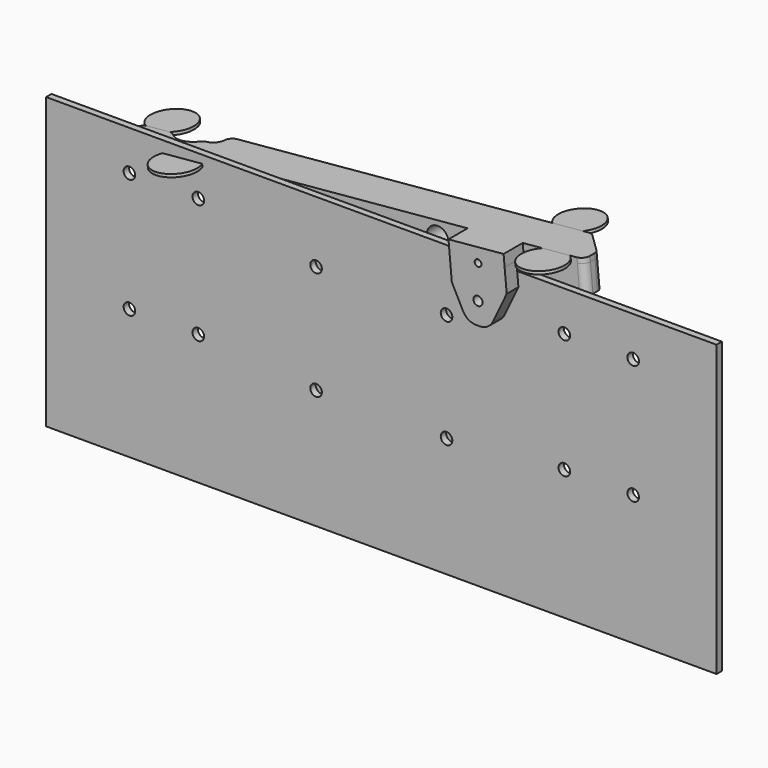
from build123d import *

# Parameters (mm, degrees)
F0_R          = 1.5875
F1_DEPTH      = 15.24
F1_DEPTH_BACK = 7.62
F2_DEPTH      = 2.4892
F3_DEPTH      = 25.4
F3_DEPTH_BACK = 0.762
F4_R          = 5.08
F5_R          = 1.7705235874
F6_DEPTH      = 26.9611633365
F7_W          = 234.95
F7_H          = 101.6
F7_R          = 2.032
F7_R_2        = 1.651
F8_DEPTH      = 2.3622
F10_DEPTH     = 114.7801239931
F11_W         = 54.61
F11_H         = 50.8
F12_DEPTH     = 25.4
F14_R         = 1.7705235874
F15_DEPTH     = 25.4
F16_R         = 3.302
F17_DEPTH     = 25.4
F18_SIZE      = 8.89
F19_R         = 1.1811
F20_DEPTH     = 48.26
F21_T4_DEPTH  = 12.1179471252
F21_S5_R      = 1.1811
F21_T6_DEPTH  = 8
F21_T11_DEPTH = 12.1179471252
F21_S12_R     = 1.1811
F21_T13_DEPTH = 8
F22_R         = 2.54
F23_R         = 7.62
F24_DEPTH     = 1.016
F25_R         = 3.7728074262
F25_R_2       = 2.7641232058
F26_DEPTH     = 28.2579587291


# Not quite as in the source:
# - a fillet or chamfer that OpenCascade refuses, or shapes differently, is made with other operations: its cross-section is extruded or revolved along the edge and cut away or added


with BuildPart() as f1:
    # F0 (on Front) → F1 (new body, two sides)
    with BuildSketch(Plane.XZ) as f1_sk:
        Polygon((-9.9150021419, 10.8382269042), (-131.9738921994, 3.3727853757), (-131.6879499686, 0.2364539576), (-9.1841964381, 2.8224508396), align=None)
        Polygon((-10.3522961262, 15.6346462997), (-132.08, 4.5366191606), (-131.9738921994, 3.3727853757), (-9.9150021419, 10.8382269042), align=None)
        Polygon((8.9584602173, 17.3952257829), (-10.3522961262, 15.6346462997), (-9.9150021419, 10.8382269042), (-0.3070324239, 11.4258755065), (9.3269835997, 13.3531104945), align=None)
        Polygon((-0.3070324239, 11.4258755065), (-9.9150021419, 10.8382269042), (-9.1841964381, 2.8224508396), (-3.81, -7.62), (3.81, -7.62), (10.047620121, 5.4488741869), (9.3269835997, 13.3531104945), align=None)
        Circle(F0_R, mode=Mode.SUBTRACT)
        Polygon((30.6387240807, 17.6164137534), (9.3269835997, 13.3531104945), (10.047620121, 5.4488741869), (31.5177794949, 7.97457419), align=None)
        Polygon((30.48, 19.3573644332), (8.9584602173, 17.3952257829), (9.3269835997, 13.3531104945), (30.6387240807, 17.6164137534), align=None)
    extrude(amount=-F1_DEPTH)
    extrude(f1_sk.sketch, amount=F1_DEPTH_BACK)

    # F0 (on Front) → F2 (cut)
    with BuildSketch(Plane.XZ):
        Polygon((-9.9150021419, 10.8382269042), (-131.9738921994, 3.3727853757), (-131.6879499686, 0.2364539576), (-9.1841964381, 2.8224508396), align=None)
        Polygon((-0.3070324239, 11.4258755065), (-9.9150021419, 10.8382269042), (-9.1841964381, 2.8224508396), (-3.81, -7.62), (3.81, -7.62), (10.047620121, 5.4488741869), (9.3269835997, 13.3531104945), align=None)
        Circle(F0_R, mode=Mode.SUBTRACT)
        Polygon((30.6387240807, 17.6164137534), (9.3269835997, 13.3531104945), (10.047620121, 5.4488741869), (31.5177794949, 7.97457419), align=None)
    extrude(amount=F2_DEPTH, mode=Mode.SUBTRACT)

    # F0 (on Front) → F3 (cut, two sides)
    with BuildSketch(Plane.XZ) as f3_sk:
        Polygon((-9.9150021419, 10.8382269042), (-131.9738921994, 3.3727853757), (-131.6879499686, 0.2364539576), (-9.1841964381, 2.8224508396), align=None)
        Polygon((-10.3522961262, 15.6346462997), (-132.08, 4.5366191606), (-131.9738921994, 3.3727853757), (-9.9150021419, 10.8382269042), align=None)
        Polygon((30.6387240807, 17.6164137534), (9.3269835997, 13.3531104945), (10.047620121, 5.4488741869), (31.5177794949, 7.97457419), align=None)
        Polygon((30.48, 19.3573644332), (8.9584602173, 17.3952257829), (9.3269835997, 13.3531104945), (30.6387240807, 17.6164137534), align=None)
    extrude(amount=F3_DEPTH, mode=Mode.SUBTRACT)
    extrude(f3_sk.sketch, amount=-F3_DEPTH_BACK, mode=Mode.SUBTRACT)

    # F4
    f4_edges = [f1.edges().sort_by_distance(p)[0] for p in [
        (-3.81, 7.62, -7.62),
        (-3.81, -5.0546, -7.62),
        (3.81, -5.0546, -7.62),
        (3.81, 7.62, -7.62),
    ]]
    fillet(f4_edges, radius=F4_R)

    # F5 (on face) → F6 (cut, through all)
    with BuildSketch(Plane(origin=(-1.4990148259, 0, 16.441808129), x_dir=(0.9958696626, 0, 0.0907943565), z_dir=(-0.0907943565, 0, 0.9958696626))):
        with Locations((-124.7725656148, 5.08)):
            Circle(F5_R)
    extrude(amount=-F6_DEPTH, mode=Mode.SUBTRACT)

    # F9 (on face) → F10 (cut, through all)
    with BuildSketch(Plane(origin=(-1.4990148259, 0, 16.441808129), x_dir=(0.9958696626, 0, 0.0907943565), z_dir=(-0.0907943565, 0, 0.9958696626))):
        with BuildLine():
            Line((-120.7187174998, 15.24), (-131.1225656148, 15.24))
            Line((-131.1225656148, 15.24), (-131.1225656148, 9.652))
            Line((-131.1225656148, 9.652), (-119.7527028025, 9.652))
            ThreePointArc((-119.7527028025, 9.652), (-120.8660431523, 12.337032401), (-120.7187174998, 15.24))
        make_face()
        with BuildLine():
            ThreePointArc((-107.9984137298, 15.24), (-114.3585656148, 20.066), (-120.7187174998, 15.24))
            Line((-120.7187174998, 15.24), (-107.9984137298, 15.24))
        make_face()
        with BuildLine():
            Line((-107.9984137298, 15.24), (-120.7187174998, 15.24))
            ThreePointArc((-120.7187174998, 15.24), (-120.8660431523, 12.337032401), (-119.7527028025, 9.652))
            Line((-119.7527028025, 9.652), (-108.9644284271, 9.652))
            ThreePointArc((-108.9644284271, 9.652), (-108.0642944899, 11.4632586445), (-107.7545656148, 13.462))
            ThreePointArc((-107.7545656148, 13.462), (-107.8158116439, 14.3593218351), (-107.9984137298, 15.24))
        make_face()
        with BuildLine():
            Line((-104.2188858955, 15.24), (-107.9984137298, 15.24))
            ThreePointArc((-107.9984137298, 15.24), (-107.8158116439, 14.3593218351), (-107.7545656148, 13.462))
            ThreePointArc((-107.7545656148, 13.462), (-108.0642944899, 11.4632586445), (-108.9644284271, 9.652))
            Line((-108.9644284271, 9.652), (-107.7748858955, 9.652))
            ThreePointArc((-107.7748858955, 9.652), (-105.2604141816, 10.6935282861), (-104.2188858955, 13.208))
            Line((-104.2188858955, 13.208), (-104.2188858955, 15.24))
        make_face()
        with BuildLine():
            Line((-108.9644284271, 9.652), (-119.7527028025, 9.652))
            ThreePointArc((-119.7527028025, 9.652), (-114.3585656148, 6.858), (-108.9644284271, 9.652))
        make_face()
    extrude(amount=-F10_DEPTH, mode=Mode.SUBTRACT)

    # F14 (on offset) → F15 (cut)
    with BuildSketch(Plane(origin=(-1.2683971604, 0, 13.9122991861), x_dir=(0.9958696626, 0, 0.0907943565), z_dir=(-0.0907943565, 0, 0.9958696626))):
        Polygon((-128.5853867925, 5.08), (-126.6789762037, 1.778), (-122.8661550259, 1.778), (-120.9597444371, 5.08), (-122.8661550259, 8.382), (-126.6789762037, 8.382), align=None)
        with Locations((-124.7725656148, 5.08)):
            Circle(F14_R, mode=Mode.SUBTRACT)
    extrude(amount=-F15_DEPTH, mode=Mode.SUBTRACT)

    # F16 (on offset) → F17 (cut)
    with BuildSketch(Plane(origin=(-1.2683971604, 0, 13.9122991861), x_dir=(0.9958696626, 0, 0.0907943565), z_dir=(-0.0907943565, 0, 0.9958696626))):
        with Locations((25.146, 5.334)):
            Circle(F16_R)
    extrude(amount=-F17_DEPTH, mode=Mode.SUBTRACT)

    # F18
    f18_edges = [f1.edges().sort_by_distance(p)[0] for p in [
        (30.99889, 15.24, 13.665969),
    ]]
    chamfer(f18_edges, length=F18_SIZE)

    # F19 (on face) → F20 (cut)
    with BuildSketch(Plane.XZ.offset(7.62)):
        with Locations((0, 11.684)):
            Circle(F19_R)
    extrude(amount=-F20_DEPTH, mode=Mode.SUBTRACT)

    # F21: fillet of radius 0.762 on 2 edges, made by hand


with BuildPart() as f8:
    # F7 (on Front) → F8 (new body)
    with BuildSketch(Plane.XZ):
        with Locations((-38.1, -40.64)):
            Rectangle(F7_W, F7_H)
        with Locations((-126.365, -45.72)):
            Circle(F7_R, mode=Mode.SUBTRACT)
        with Locations((-102.235, -45.72)):
            Circle(F7_R, mode=Mode.SUBTRACT)
        with Locations((-60.96, -49.53)):
            Circle(F7_R, mode=Mode.SUBTRACT)
        with Locations((-15.24, -49.53)):
            Circle(F7_R, mode=Mode.SUBTRACT)
        with Locations((26.035, -45.72)):
            Circle(F7_R, mode=Mode.SUBTRACT)
        with Locations((50.165, -45.72)):
            Circle(F7_R, mode=Mode.SUBTRACT)
        with Locations((-126.365, -3.81)):
            Circle(F7_R, mode=Mode.SUBTRACT)
        with Locations((-102.235, -3.81)):
            Circle(F7_R, mode=Mode.SUBTRACT)
        with Locations((-60.96, -11.43)):
            Circle(F7_R, mode=Mode.SUBTRACT)
        with Locations((-15.24, -11.43)):
            Circle(F7_R, mode=Mode.SUBTRACT)
        Circle(F7_R_2, mode=Mode.SUBTRACT)
        with Locations((26.035, -3.81)):
            Circle(F7_R, mode=Mode.SUBTRACT)
        with Locations((50.165, -3.81)):
            Circle(F7_R, mode=Mode.SUBTRACT)
    extrude(amount=F8_DEPTH)

    # F11 (on face) → F12 (join)
    with BuildSketch(Plane.XZ):
        with Locations((-38.1, -28.448)):
            Rectangle(F11_W, F11_H)
    extrude(amount=-F12_DEPTH)


with BuildPart() as f21_tool2:
    # F21_s3 → F21_t4 (new body)
    with BuildSketch(Plane(origin=(13.4045259726, 0, 2.6815059668), x_dir=(0, 1, 0), z_dir=(-0.9805722233, 0, -0.1961583925))):
        with BuildLine():
            ThreePointArc((0, -10.5021231349), (-0.2231846327, -11.0409385022), (-0.762, -11.2641231349))
            Line((-0.762, -11.2641231349), (0, -11.2641231349))
            Line((0, -11.2641231349), (0, -10.5021231349))
        make_face()
    extrude(amount=F21_T4_DEPTH)

    # F21_s5 → F21_t6 (cut, symmetric)
    with BuildSketch(Plane.XZ.offset(0.4)):
        with Locations((0, 11.684)):
            Circle(F21_S5_R)
    extrude(amount=F21_T6_DEPTH, both=True, mode=Mode.SUBTRACT)

    split(bisect_by=Plane(origin=(10.4574750432, 0, 0.9534176539), x_dir=(0, 1, 0), z_dir=(-0.9958696626, 0, -0.0907943565)), keep=Keep.TOP)


with BuildPart() as f1_1:
    add(f1.part)

    # F21_t1: union F21_tool2
    add(f21_tool2.part)


with BuildPart() as f21_tool9:
    # F21_s10 → F21_t11 (new body)
    with BuildSketch(Plane(origin=(13.4045259726, 0, 2.6815059668), x_dir=(0, 1, 0), z_dir=(-0.9805722233, 0, -0.1961583925))):
        with BuildLine():
            ThreePointArc((-2.4892, -10.5021231349), (-2.2660153673, -11.0409385022), (-1.7272, -11.2641231349))
            Line((-1.7272, -11.2641231349), (-2.4892, -11.2641231349))
            Line((-2.4892, -11.2641231349), (-2.4892, -10.5021231349))
        make_face()
    extrude(amount=F21_T11_DEPTH)

    # F21_s12 → F21_t13 (cut, symmetric)
    with BuildSketch(Plane.XZ.offset(2.1)):
        with Locations((0, 11.684)):
            Circle(F21_S12_R)
    extrude(amount=F21_T13_DEPTH, both=True, mode=Mode.SUBTRACT)

    split(bisect_by=Plane(origin=(10.4574750432, 0, 0.9534176539), x_dir=(0, 1, 0), z_dir=(-0.9958696626, 0, -0.0907943565)), keep=Keep.TOP)


with BuildPart() as f1_2:
    add(f1_1.part)

    # F21_t8: union F21_tool9
    add(f21_tool9.part)

    # F22
    f22_edges = [f1_2.edges().sort_by_distance(p)[0] for p in [
        (30.99889, 0.762, 13.665969),
        (30.99889, 6.35, 13.665969),
        (22.156177, 15.24, 12.742892),
        (-131.883975, 9.652, 2.386537),
        (-120.52498, 9.652, 3.022969),
        (-109.747018, 9.652, 3.626846),
        (-105.006011, 15.24, 3.89248),
        (-131.883975, 0.762, 2.386537),
    ]]
    fillet(f22_edges, radius=F22_R)

    # F23 (on face) → F24 (join)
    with BuildSketch(Plane(origin=(-1.4990148259, 0, 16.441808129), x_dir=(0.9958696626, 0, 0.0907943565), z_dir=(-0.0907943565, 0, 0.9958696626))):
        with Locations((14.6784631455, 20.6369586291)):
            Circle(F23_R)
        with Locations((22.310359779, -5.1038903915)):
            Circle(F23_R)
        with Locations((-106.7618331113, -5.4179092716)):
            Circle(F23_R)
        with Locations((-125.0981798966, 15.988830362)):
            Circle(F23_R)
    extrude(amount=-F24_DEPTH)

    # F25 (on Front) → F26 (cut, through all)
    with BuildSketch(Plane.XZ):
        with Locations((-20.849423483, 9.2049865052)):
            Circle(F25_R)
        with Locations((-72.0916762948, 5.7735857554)):
            Circle(F25_R_2)
    extrude(amount=-F26_DEPTH, mode=Mode.SUBTRACT)


solid = Compound([f8.part, f1_2.part])
